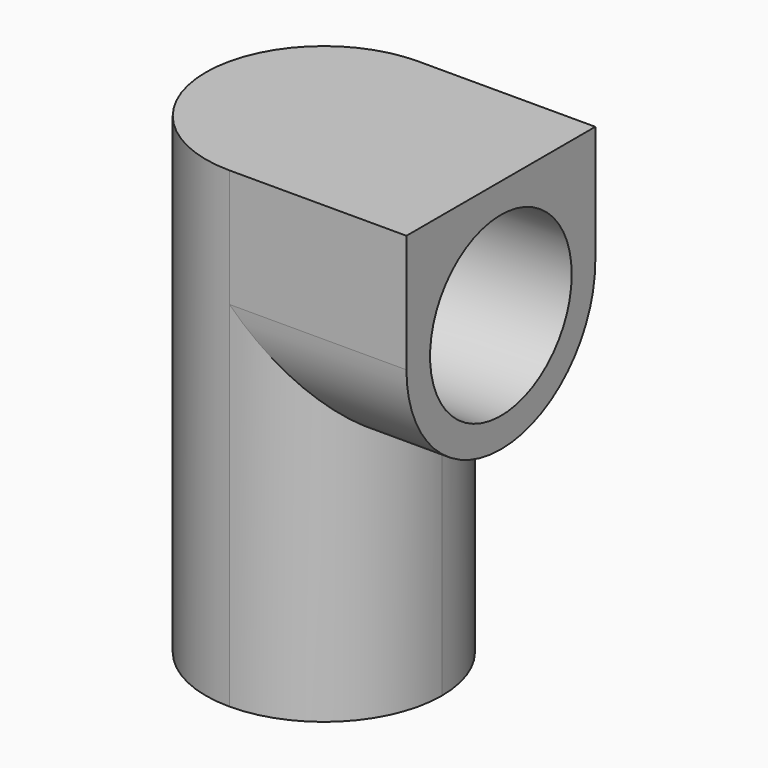
from build123d import *

# Parameters (mm, degrees)
F1_DEPTH = 40
F2_R     = 15
F3_DEPTH = 40
F4_R     = 12.75
F5_DEPTH = 30
F6_R     = 19.99999
F7_R     = 19.99999


# Not quite as in the source:
# - a fillet or chamfer is up to 0.001 mm smaller than in the source, because OpenCascade refuses the exact size


with BuildPart() as f1:
    # F0 (on Front) → F1 (new body)
    with BuildSketch(Plane.XZ):
        Polygon((0, -40), (0, 0), (10, 0), (10, 40), (-40, 40), (-40, -40), align=None)
    extrude(amount=-F1_DEPTH)

    # F2 (on face) → F3 (cut)
    with BuildSketch(Plane.YZ.offset(10)):
        with Locations((20, 20)):
            Circle(F2_R)
    extrude(amount=-F3_DEPTH, mode=Mode.SUBTRACT)

    # F4 (on face) → F5 (cut)
    with BuildSketch(Plane(origin=(0, 0, -40), x_dir=(1, 0, 0), z_dir=(0, 0, -1))):
        with Locations((-20, -20)):
            Circle(F4_R)
    extrude(amount=-F5_DEPTH, mode=Mode.SUBTRACT)

    # F6 (radius 20 in the source; OpenCascade refuses exactly that, so slightly less here)
    f6_edges = [f1.edges().sort_by_distance(p)[0] for p in [
        (-40, 40, 0),
        (-40, 0, 0),
    ]]
    fillet(f6_edges, radius=F6_R)

    # F7 (radius 20 in the source; OpenCascade refuses exactly that, so slightly less here)
    f7_edges = [f1.edges().sort_by_distance(p)[0] for p in [
        (0, 0, -20),
        (0, 40, -20),
        (5, 0, 0),
        (5, 40, 0),
    ]]
    fillet(f7_edges, radius=F7_R)


solid = f1.part
